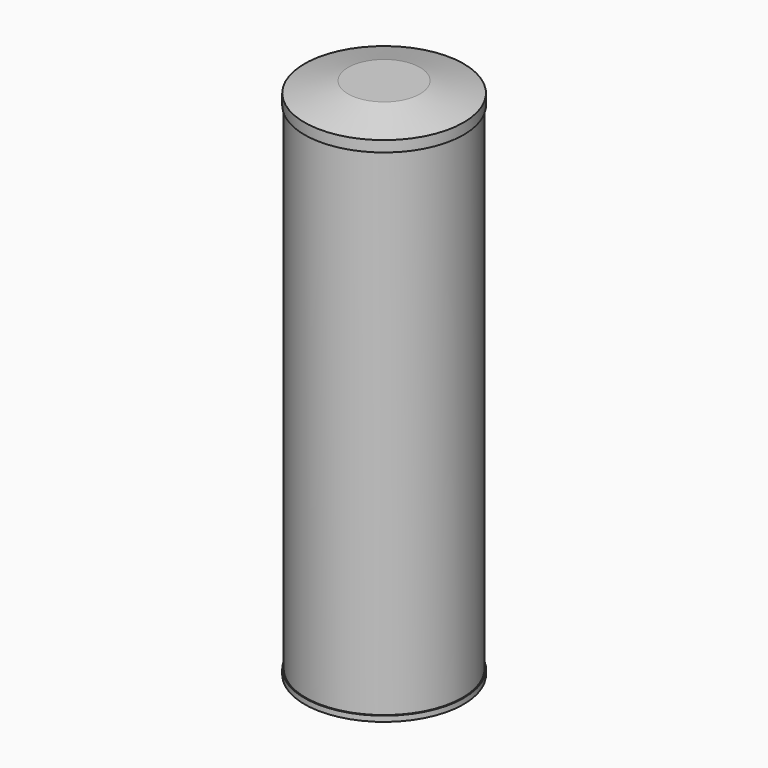
from build123d import *

# Parameters (mm, degrees)
F0_R     = 185.42
F1_DEPTH = 12.7
F2_R     = 182.88
F2_R_2   = 181.61
F3_DEPTH = 1181.1
F4_R     = 185.42
F5_DEPTH = 25.4
F6_SIZE2 = 25.39999
F6_SIZE  = 101.59999
F7_R     = 185.42
F7_R_2   = 182.88
F8_DEPTH = 25.4


# Not quite as in the source:
# - a fillet or chamfer is up to 0.001 mm smaller than in the source, because OpenCascade refuses the exact size


with BuildPart() as f1:
    # F0 (on Top) → F1 (new body)
    with BuildSketch(Plane.XY):
        Circle(F0_R)
    extrude(amount=F1_DEPTH)

    # F2 (on face) → F3 (join)
    with BuildSketch(Plane.XY.offset(12.7)):
        Circle(F2_R)
        Circle(F2_R_2, mode=Mode.SUBTRACT)
    extrude(amount=F3_DEPTH)

    # F4 (on face) → F5 (join)
    with BuildSketch(Plane.XY.offset(1193.8)):
        Circle(F4_R)
    extrude(amount=F5_DEPTH)

    # F6 (size 101.6 and 25.4 in the source; OpenCascade refuses exactly that, so slightly less here)
    f6_edges = [f1.edges().sort_by_distance(p)[0] for p in [
        (-185.42, 0, 1219.2),
    ]]
    f6_side = f1.faces().sort_by_distance((0, 0, 1219.2))[0]
    chamfer(f6_edges, length=F6_SIZE, length2=F6_SIZE2, reference=f6_side)

    # F7 (on face) → F8 (join)
    with BuildSketch(Plane(origin=(0, 0, 1193.8), x_dir=(1, 0, 0), z_dir=(0, 0, -1))):
        Circle(F7_R)
        Circle(F7_R_2, mode=Mode.SUBTRACT)
    extrude(amount=F8_DEPTH)


solid = f1.part
